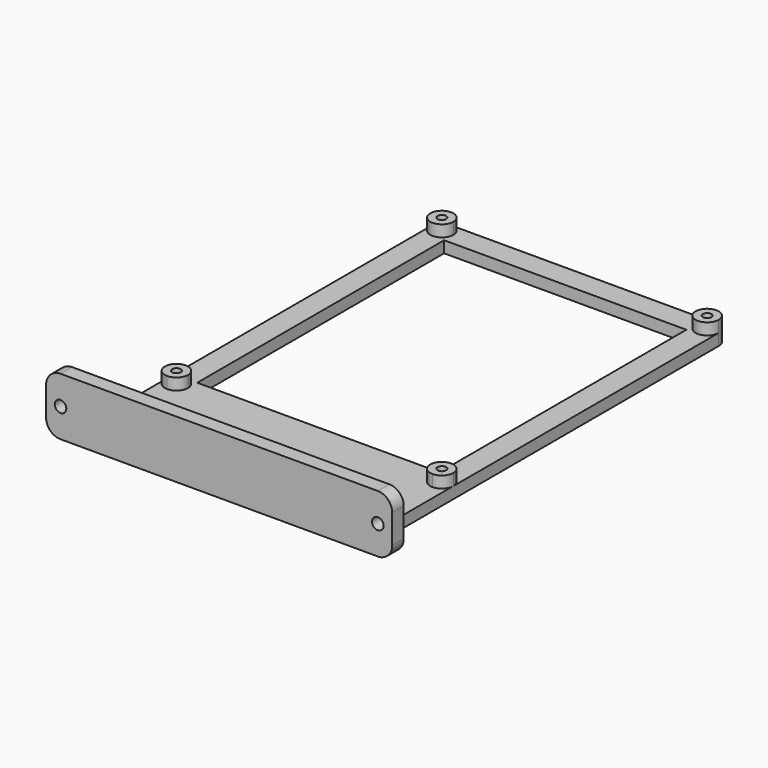
from build123d import *

# Parameters (mm, degrees)
F0_W      = 100
F0_H      = 122.999
F0_R      = 1.5
F0_W_2    = 84
F0_H_2    = 106.999
F1_DEPTH  = 4
F2_R      = 1.5
F3_DEPTH  = 4
F4_W      = 100
F4_H      = 4
F5_DEPTH  = 30
F7_DEPTH  = 20
F8_R      = 4.99999
F9_R      = 3.9999
F10_R     = 2
F11_DEPTH = 10


# Not quite as in the source:
# - a fillet or chamfer is up to 0.001 mm smaller than in the source, because OpenCascade refuses the exact size


with BuildPart() as f1:
    # F0 (on Top) → F1 (new body)
    with BuildSketch(Plane.XY):
        Rectangle(F0_W, F0_H)
        with Locations((-46, -57.4995)):
            Circle(F0_R, mode=Mode.SUBTRACT)
        with Locations((46, -57.4995)):
            Circle(F0_R, mode=Mode.SUBTRACT)
        with Locations((-46, 57.4995)):
            Circle(F0_R, mode=Mode.SUBTRACT)
        Rectangle(F0_W_2, F0_H_2, mode=Mode.SUBTRACT)
        with Locations((46, 57.4995)):
            Circle(F0_R, mode=Mode.SUBTRACT)
    extrude(amount=F1_DEPTH)

    # F2 (on face) → F3 (join)
    with BuildSketch(Plane.XY.offset(4)):
        with BuildLine():
            ThreePointArc((-42, 57.4995), (-43.1715728523, 60.3279271017), (-45.999999935, 61.4995))
            ThreePointArc((-45.999999935, 61.4995), (-48.8284271017, 60.3279271477), (-50, 57.4995))
            ThreePointArc((-50, 57.4995), (-46, 53.4995), (-42, 57.4995))
        make_face()
        with Locations((-46, 57.4995)):
            Circle(F2_R, mode=Mode.SUBTRACT)
        with BuildLine():
            ThreePointArc((46, 61.4995), (43.1715728753, 54.6710728753), (50, 57.4995))
            ThreePointArc((50, 57.4995), (48.8284271247, 60.3279271247), (46, 61.4995))
        make_face()
        with Locations((46, 57.4995)):
            Circle(F2_R, mode=Mode.SUBTRACT)
        with BuildLine():
            ThreePointArc((45.9999999936, -61.4995), (48.8284271225, -60.327927127), (50, -57.4995))
            ThreePointArc((50, -57.4995), (43.1715728775, -54.671072873), (45.9999999936, -61.4995))
        make_face()
        with Locations((46, -57.4995)):
            Circle(F2_R, mode=Mode.SUBTRACT)
        with BuildLine():
            ThreePointArc((-50, -57.4995), (-48.8284271247, -60.3279271247), (-46, -61.4995))
            ThreePointArc((-46, -61.4995), (-43.1715728753, -60.3279271247), (-42, -57.4995))
            ThreePointArc((-42, -57.4995), (-46, -53.4995), (-50, -57.4995))
        make_face()
        with Locations((-46, -57.4995)):
            Circle(F2_R, mode=Mode.SUBTRACT)
    extrude(amount=F3_DEPTH)

    # F4 (on face) → F5 (join)
    with BuildSketch(Plane.XZ.offset(61.4995)):
        with Locations((0, 2)):
            Rectangle(F4_W, F4_H)
    extrude(amount=F5_DEPTH)

    # F6 (on face) → F7 (join)
    with BuildSketch(Plane(origin=(0, 0, 0), x_dir=(1, 0, 0), z_dir=(0, 0, -1))):
        Polygon((50, 91.4995), (60, 91.4995), (60, 96.4995), (-50, 96.4995), (-60, 96.4995), (-60, 91.4995), (-50, 91.4995), align=None)
    extrude(amount=-F7_DEPTH)

    # F8 (radius 5 in the source; OpenCascade refuses exactly that, so slightly less here)
    f8_edges = [f1.edges().sort_by_distance(p)[0] for p in [
        (-60, -93.9995, 20),
        (-60, -93.9995, 0),
        (60, -93.9995, 0),
        (60, -93.9995, 20),
        (50, -91.4995, 2),
        (-50, -91.4995, 2),
    ]]
    fillet(f8_edges, radius=F8_R)

    # F9 (radius 4 in the source; OpenCascade refuses exactly that, so slightly less here)
    f9_edges = [f1.edges().sort_by_distance(p)[0] for p in [
        (50, 61.4995, 2),
        (-50, 61.4995, 2),
    ]]
    fillet(f9_edges, radius=F9_R)

    # F10 (on face) → F11 (cut)
    with BuildSketch(Plane(origin=(0, -91.4995, 0), x_dir=(-1, 0, 0), z_dir=(0, 1, 0))):
        with Locations((55, 10)):
            Circle(F10_R)
        with Locations((-55, 10)):
            Circle(F10_R)
    extrude(amount=-F11_DEPTH, mode=Mode.SUBTRACT)


solid = f1.part
